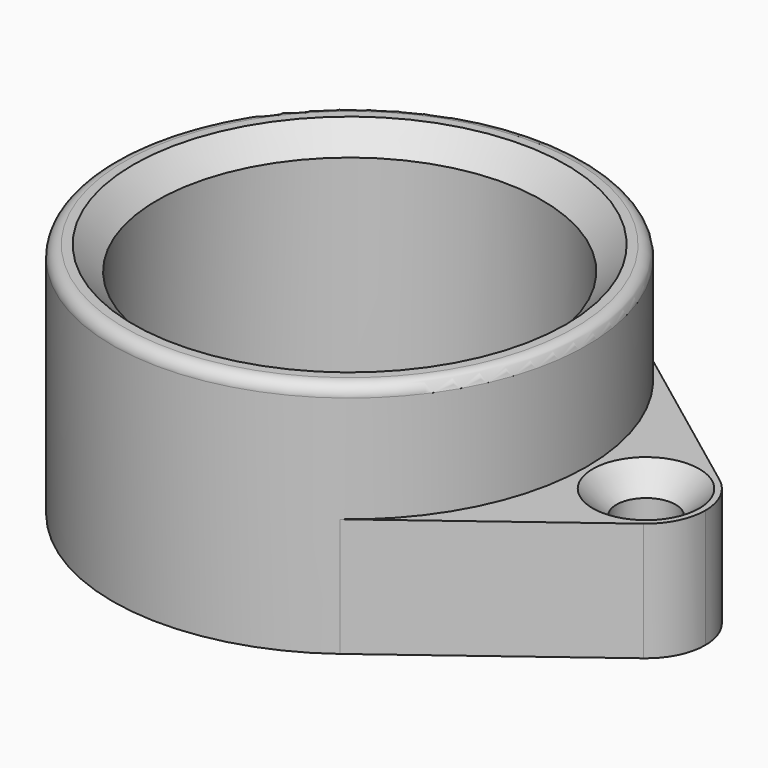
from build123d import *

# Parameters (mm, degrees)
F0_R     = 41.275
F0_R_2   = 6.35
F1_DEPTH = 25.4
F2_DEPTH = 50.8
F3_R     = 2.54
F4_SIZE  = 5.08


# Not quite as in the source:
# - a feature names something its author has since deleted; it is built from what else it names


with BuildPart() as f1:
    # F0 (on Top) → F1 (new body)
    with BuildSketch(Plane.XY):
        with BuildLine():
            ThreePointArc((30.48, -40.64), (45.4369013028, -22.7184506514), (50.8, 0))
            ThreePointArc((50.8, 0), (45.4369013028, 22.7184506514), (30.48, 40.64))
            ThreePointArc((30.48, 40.64), (-50.8, 0), (30.48, -40.64))
        make_face()
        Circle(F0_R, mode=Mode.SUBTRACT)
        with BuildLine():
            ThreePointArc((71.12, 10.16), (57.8203873372, 11.3592253257), (50.8, 0))
            ThreePointArc((50.8, 0), (57.8203873372, -11.3592253257), (71.12, -10.16))
            ThreePointArc((71.12, -10.16), (74.8592253257, -5.6796126628), (76.2, 0))
            ThreePointArc((76.2, 0), (74.8592253257, 5.6796126628), (71.12, 10.16))
        make_face()
        with Locations((63.5, 0)):
            Circle(F0_R_2, mode=Mode.SUBTRACT)
        with BuildLine():
            ThreePointArc((71.12, -10.16), (57.8203873372, -11.3592253257), (50.8, 0))
            ThreePointArc((50.8, 0), (45.4369013028, -22.7184506514), (30.48, -40.64))
            Line((30.48, -40.64), (71.12, -10.16))
        make_face()
        with BuildLine():
            ThreePointArc((30.48, 40.64), (45.4369013028, 22.7184506514), (50.8, 0))
            ThreePointArc((50.8, 0), (57.8203873372, 11.3592253257), (71.12, 10.16))
            Line((71.12, 10.16), (30.48, 40.64))
        make_face()
    extrude(amount=F1_DEPTH)

    # F0 (on Top) → F2 (join)
    with BuildSketch(Plane.XY):
        with BuildLine():
            ThreePointArc((30.48, -40.64), (45.4369013028, -22.7184506514), (50.8, 0))
            ThreePointArc((50.8, 0), (45.4369013028, 22.7184506514), (30.48, 40.64))
            ThreePointArc((30.48, 40.64), (-50.8, 0), (30.48, -40.64))
        make_face()
        Circle(F0_R, mode=Mode.SUBTRACT)
    extrude(amount=F2_DEPTH)

    # F3
    f3_edges = [f1.edges().sort_by_distance(p)[0] for p in [
        (-30.48, 40.64, 50.8),
    ]]
    fillet(f3_edges, radius=F3_R)

    # F4
    f4_edges = [f1.edges().sort_by_distance(p)[0] for p in [
        (-41.275, 0, 50.8),
        (57.15, 0, 25.4),
    ]]
    chamfer(f4_edges, length=F4_SIZE)


solid = f1.part
